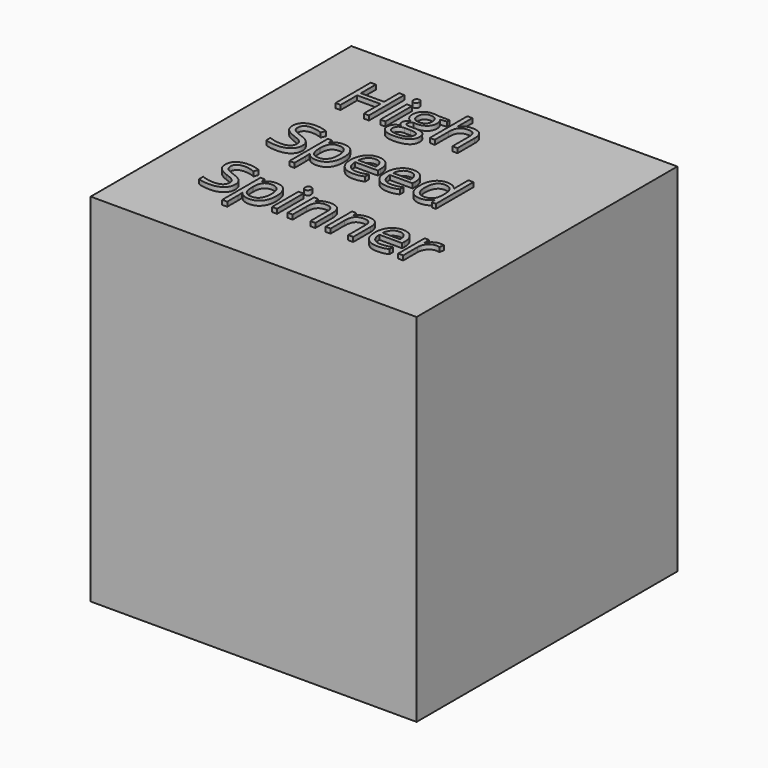
from build123d import *

# Parameters (mm, degrees)
F0_W         = 1828.8
F0_H         = 1828.8
F1_DEPTH     = 2000
F2_TEXT_SIZE = 346.7872685383
F3_DEPTH     = 25.4


# Not quite as in the source:
# - Text() gives the source's letters only with a copy of the font that has no kerning and outlines rounded to 1/6400 em; it was checked with that copy


with BuildPart() as f1:
    # F0 (on Top) → F1 (new body)
    with BuildSketch(Plane.XY):
        Rectangle(F0_W, F0_H)
    extrude(amount=F1_DEPTH)

    # F2 (on face) → F3 (join)
    with BuildSketch(Plane.XY.offset(2000)):
        with Locations((-635, 410.7131666524)):
            Text('High', F2_TEXT_SIZE, font='Open Sans', text_align=(TextAlign.LEFT, TextAlign.BOTTOM))
        with Locations((-635, -60.9175185596)):
            Text('Speed', F2_TEXT_SIZE, font='Open Sans', text_align=(TextAlign.LEFT, TextAlign.BOTTOM))
        with Locations((-635, -532.5482037717)):
            Text('Spinner', F2_TEXT_SIZE, font='Open Sans', text_align=(TextAlign.LEFT, TextAlign.BOTTOM))
    extrude(amount=F3_DEPTH)


solid = f1.part
